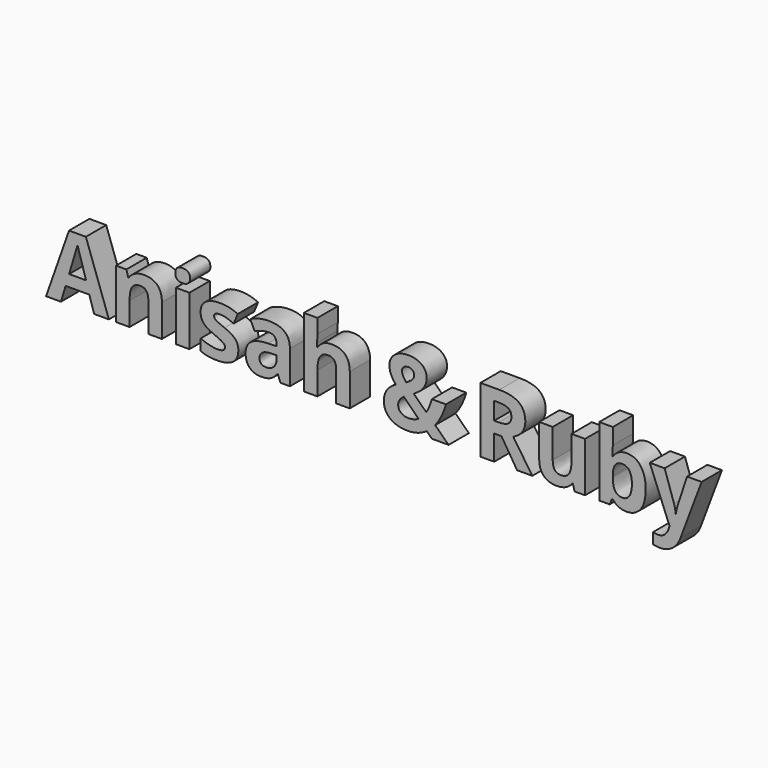
from build123d import *

# Parameters (mm, degrees)
F0_TEXT_SIZE = 60.9395197696
F1_DEPTH     = 17.018


# Not quite as in the source:
# - Text() gives the source's letters only with a copy of the font that has no kerning and outlines rounded to 1/6400 em; it was checked with that copy


with BuildPart() as f1:
    # F0 (on Front) → F1 (new body)
    with BuildSketch(Plane.XZ):
        with Locations((-76.507255435, 11.2456455827)):
            Text('Anisah & Ruby', F0_TEXT_SIZE, font='Open Sans', font_style=FontStyle.BOLD, text_align=(TextAlign.LEFT, TextAlign.BOTTOM))
    extrude(amount=F1_DEPTH)


solid = f1.part
